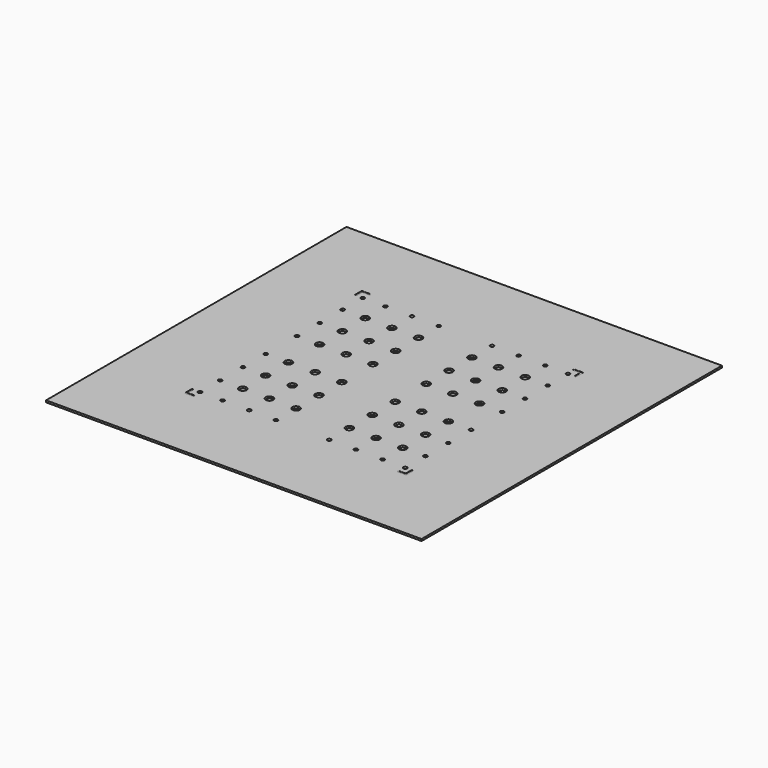
from build123d import *

# Parameters (mm, degrees)
F0_W     = 200
F0_H     = 200
F1_DEPTH = 1
F3_D     = 4
F5_D     = 2
F7_DEPTH = 0.1
F8_R     = 0.49999


# Not quite as in the source:
# - a fillet or chamfer is up to 0.001 mm smaller than in the source, because OpenCascade refuses the exact size


with BuildPart() as f1:
    # F0 (on Top) → F1 (new body)
    with BuildSketch(Plane.XY):
        Rectangle(F0_W, F0_H)
    extrude(amount=F1_DEPTH)

    # F3 (through all)
    with Locations(Plane.XY.offset(1)):
        with Locations((-42.6, 40.75), (-28.4, 40.75), (-14.2, 40.75), (14.2, 40.75), (28.4, 40.75), (42.6, 40.75), (-42.6, 25.55), (-28.4, 25.55), (-14.2, 25.55), (14.2, 25.55), (28.4, 25.55), (42.6, 25.55), (42.6, 10.35), (28.4, 10.35), (14.2, 10.35), (-14.2, 10.35), (-28.4, 10.35), (-42.6, 10.35), (-42.6, -10.35), (-28.4, -10.35), (-14.2, -10.35), (14.2, -10.35), (28.4, -10.35), (42.6, -10.35), (42.6, -25.55), (28.4, -25.55), (14.2, -25.55), (-14.2, -25.55), (-28.4, -25.55), (-42.6, -25.55), (-42.6, -40.75), (-28.4, -40.75), (-14.2, -40.75), (14.2, -40.75), (28.4, -40.75), (42.6, -40.75)):
            Hole(F3_D / 2)

    # F5 (through all)
    with Locations(Plane.XY.offset(1)):
        with Locations((-54.65, 54.2), (-42.6, 54.2), (-28.4, 54.2), (-14.2, 54.2), (14.2, 54.2), (28.4, 54.2), (42.6, 54.2), (54.65, 54.2), (54.65, 40.75), (54.65, 25.55), (54.65, 10.35), (54.65, -10.35), (54.65, -25.55), (54.65, -40.75), (54.65, -54.2), (42.6, -54.2), (28.4, -54.2), (14.2, -54.2), (-14.2, -54.2), (-28.4, -54.2), (-42.6, -54.2), (-54.65, -54.2), (-54.65, -40.75), (-54.65, -25.55), (-54.65, -10.35), (-54.65, 10.35), (-54.65, 25.55), (-54.65, 40.75)):
            Hole(F5_D / 2)

    # F6 (on face) → F7 (cut)
    with BuildSketch(Plane.XY.offset(1)):
        Polygon((-58, 59), (-59, 59), (-59, 58), (-59, 54), (-58, 54), (-58, 58), (-54, 58), (-54, 59), align=None)
        Polygon((-59, -58), (-59, -59), (-58, -59), (-54, -59), (-54, -58), (-58, -58), (-58, -54), (-59, -54), align=None)
        Polygon((58, -59), (59, -59), (59, -58), (59, -54), (58, -54), (58, -58), (54, -58), (54, -59), align=None)
        Polygon((59, 58), (59, 59), (58, 59), (54, 59), (54, 58), (58, 58), (58, 54), (59, 54), align=None)
    extrude(amount=-F7_DEPTH, mode=Mode.SUBTRACT)

    # F8 (radius 0.5 in the source; OpenCascade refuses exactly that, so slightly less here)
    f8_edges = [f1.edges().sort_by_distance(p)[0] for p in [
        (-54, 59, 0.95),
        (-54, 58, 0.95),
        (-59, 59, 0.95),
        (-59, 54, 0.95),
        (-58, 54, 0.95),
        (54, 59, 0.95),
        (54, 58, 0.95),
        (59, 59, 0.95),
        (59, 54, 0.95),
        (58, 54, 0.95),
        (59, -54, 0.95),
        (58, -54, 0.95),
        (59, -59, 0.95),
        (54, -58, 0.95),
        (54, -59, 0.95),
        (-58, -54, 0.95),
        (-59, -54, 0.95),
        (-59, -59, 0.95),
        (-54, -58, 0.95),
        (-54, -59, 0.95),
    ]]
    fillet(f8_edges, radius=F8_R)


solid = f1.part
